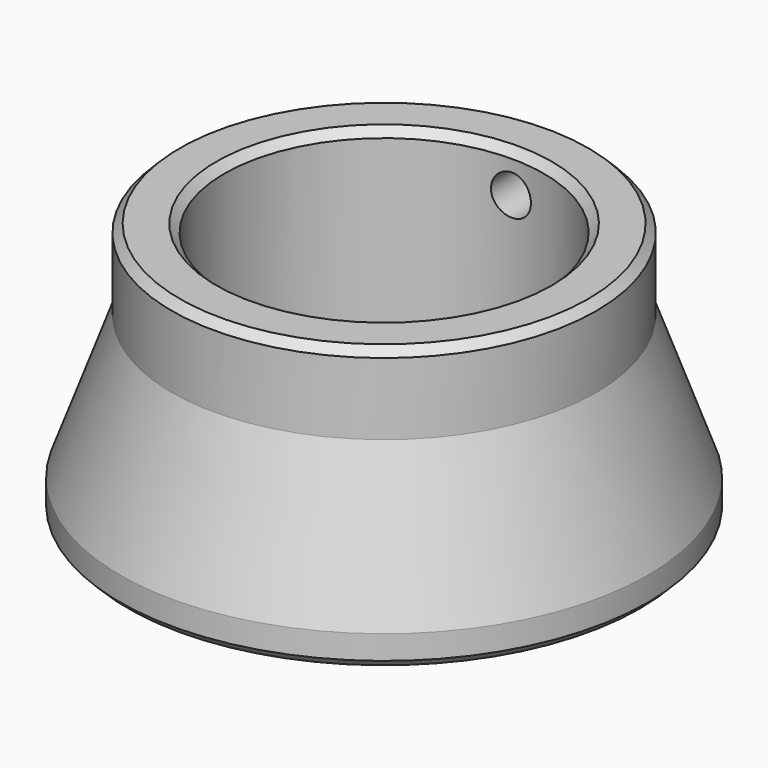
from build123d import *

# Parameters (mm, degrees)
F3_D     = 2.5
F3_DEPTH = 16.521
F4_SIZE  = 0.5


with BuildPart() as f1:
    # F0 (on Front) → F1 (revolve)
    with BuildSketch(Plane.XZ):
        Polygon((10, 16), (10, 0), (16.52, 0), (16.52, 2), (13.28, 11), (13.28, 15.774938604), (13.28, 16), align=None)
    revolve(axis=Axis((0, 0, 22.1384353936), (0, 0, 1)))

    # F3 (through all, one way)
    with BuildSketch(Plane.XZ):
        with Locations((0, 13.5)):
            Circle(F3_D / 2)
    extrude(amount=-F3_DEPTH, mode=Mode.SUBTRACT)

    # F4
    f4_edges = [f1.edges().sort_by_distance(p)[0] for p in [
        (-13.28, 0, 16),
        (-10, 0, 16),
        (-10, 0, 0),
        (-16.52, 0, 0),
    ]]
    chamfer(f4_edges, length=F4_SIZE)


solid = f1.part
